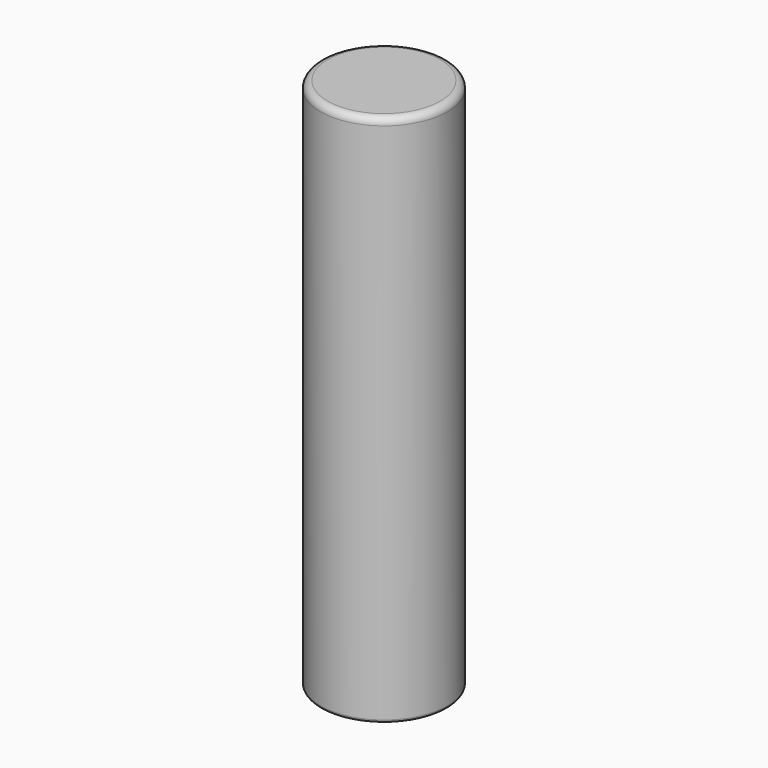
from build123d import *

# Parameters (mm, degrees)
F2_R = 2.54
F3_R = 1.01599


# Not quite as in the source:
# - a fillet or chamfer is up to 0.001 mm smaller than in the source, because OpenCascade refuses the exact size


with BuildPart() as f1:
    # F0 (on Front) → F1 (revolve)
    with BuildSketch(Plane.XZ):
        with BuildLine():
            Line((0, -21.7963978648), (0, 0))
            Line((0, 0), (-22.6568, 0))
            Line((-22.6568, 0), (-22.6568, -190.5))
            Line((-22.6568, -190.5), (-20.6248, -190.5))
            Line((-20.6248, -190.5), (-20.6248, -27.3231199056))
            ThreePointArc((-20.6248, -27.3231199056), (-20.108359218, -25.7879299854), (-18.7690455975, -24.877019343))
            add(Edge.make_bspline(
                [(-18.7690455975, -24.877019343), (-15.7267844832, -24.0260102693), (-9.2902414756, -22.325160199), (-3.2160062892, -21.9794397154), (0, -21.7963978648)],
                knots=[0.0872743239, 0.0872743239, 0.0872743239, 0.0872743239, 0.5167570197, 1, 1, 1, 1], degree=3))
        make_face()
    revolve(axis=Axis((0, 0, -10.8981989324), (0, 0, 1)))

    # F2
    f2_edges = [f1.edges().sort_by_distance(p)[0] for p in [
        (22.6568, 0, 0),
    ]]
    fillet(f2_edges, radius=F2_R)

    # F3 (radius 1.016 in the source; OpenCascade refuses exactly that, so slightly less here)
    f3_edges = [f1.edges().sort_by_distance(p)[0] for p in [
        (22.6568, 0, -190.5),
        (20.6248, 0, -190.5),
    ]]
    fillet(f3_edges, radius=F3_R)


solid = f1.part
